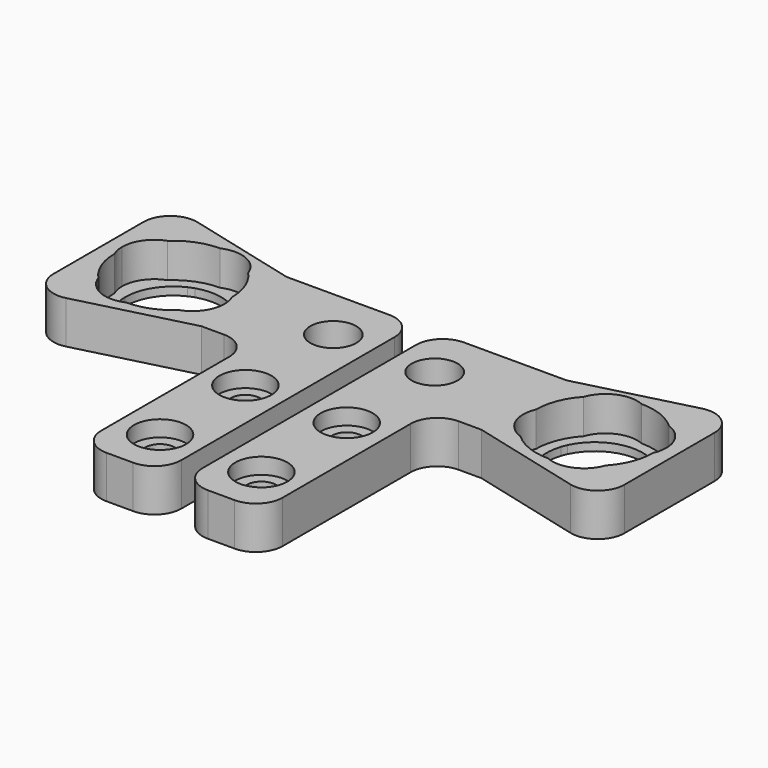
from build123d import *

# Parameters (mm, degrees)
F1_DEPTH       = 8
F2_D           = 8.6
F3_D           = 5.5
F3_CBORE_D     = 9.75
F3_CBORE_DEPTH = 3
F4_R           = 5
F5_START       = -6.5
F5_DEPTH       = 1.5


# Not quite as in the source:
# - a feature names something its author has since deleted; it is built from what else it names


with BuildPart() as f1:
    # F0 (on Top) → F1 (new body)
    with BuildSketch(Plane.XY):
        Polygon((53.5, 33), (53.5, 67), (26.25, 60), (2, 60), (2, 40), (2, 0), (17, 0), (17, 40), (26.25, 40), align=None)
        with BuildLine():
            ThreePointArc((51, 52.3979157617), (50.8736700622, 51.1731708903), (50.5, 50))
            ThreePointArc((50.5, 50), (49.7385612859, 45.978574532), (47.55966131, 42.5138888889))
            ThreePointArc((47.55966131, 42.5138888889), (44.2958315233, 39), (39.5, 39))
            ThreePointArc((39.5, 39), (35.478574532, 39.7614387141), (32.0138888889, 41.94033869))
            ThreePointArc((32.0138888889, 41.94033869), (28.5, 45.2041684767), (28.5, 50))
            ThreePointArc((28.5, 50), (29.2614387141, 54.021425468), (31.44033869, 57.4861111111))
            ThreePointArc((31.44033869, 57.4861111111), (34.7041684767, 61), (39.5, 61))
            ThreePointArc((39.5, 61), (43.521425468, 60.2385612859), (46.9861111111, 58.05966131))
            ThreePointArc((46.9861111111, 58.05966131), (49.8947250519, 55.8680262306), (51, 52.3979157617))
        make_face(mode=Mode.SUBTRACT)
    extrude(amount=-F1_DEPTH)

    # F2 (through all)
    with Locations(Plane.XY):
        with Locations((9.5, 50)):
            Hole(F2_D / 2)

    # F3 (through all)
    with Locations(Plane.XY):
        with Locations((9.5, 29.4), (9.5, 9.4)):
            CounterBoreHole(F3_D / 2, F3_CBORE_D / 2, F3_CBORE_DEPTH)

    # F4
    f4_edges = [f1.edges().sort_by_distance(p)[0] for p in [
        (17, 0, -4),
        (2, 60, -4),
        (53.5, 33, -4),
        (53.5, 67, -4),
        (17, 40, -4),
        (2, 0, -4),
    ]]
    fillet(f4_edges, radius=F4_R)

    # F0 (on Top) → F5 (join)
    with BuildSketch(Plane.XY.offset(F5_START)):
        with BuildLine():
            ThreePointArc((42.2592068472, 58.5666082888), (41.0707112049, 60), (39.5, 61))
            ThreePointArc((39.5, 61), (35.1038211036, 60.0833333333), (31.44033869, 57.4861111111))
            ThreePointArc((31.44033869, 57.4861111111), (31.104078936, 55.6547009803), (31.3454826891, 53.8083917112))
            ThreePointArc((31.3454826891, 53.8083917112), (35.9031263575, 58.25), (42.2592068472, 58.5666082888))
        make_face()
        with BuildLine():
            ThreePointArc((31.44033869, 57.4861111111), (35.1038211036, 60.0833333333), (39.5, 61))
            ThreePointArc((39.5, 61), (34.7041684767, 61), (31.44033869, 57.4861111111))
        make_face()
        with BuildLine():
            ThreePointArc((43.3083917112, 58.1545173109), (45.1547009803, 58.395921064), (46.9861111111, 58.05966131))
            ThreePointArc((46.9861111111, 58.05966131), (43.521425468, 60.2385612859), (39.5, 61))
            ThreePointArc((39.5, 61), (41.0707112049, 60), (42.2592068472, 58.5666082888))
            ThreePointArc((42.2592068472, 58.5666082888), (42.7902572011, 58.3770046885), (43.3083917112, 58.1545173109))
        make_face()
        with BuildLine():
            ThreePointArc((48.0666082888, 47.2407931528), (49.5, 48.4292887951), (50.5, 50))
            ThreePointArc((50.5, 50), (49.5833333333, 54.3961788964), (46.9861111111, 58.05966131))
            ThreePointArc((46.9861111111, 58.05966131), (45.1547009803, 58.395921064), (43.3083917112, 58.1545173109))
            ThreePointArc((43.3083917112, 58.1545173109), (47.0919538131, 54.8334498342), (48.5, 50))
            ThreePointArc((48.5, 50), (48.3909919188, 48.603481937), (48.0666082888, 47.2407931528))
        make_face()
        with BuildLine():
            ThreePointArc((46.9861111111, 58.05966131), (49.5833333333, 54.3961788964), (50.5, 50))
            ThreePointArc((50.5, 50), (50.8736700622, 51.1731708903), (51, 52.3979157617))
            ThreePointArc((51, 52.3979157617), (49.8947250519, 55.8680262306), (46.9861111111, 58.05966131))
        make_face()
        with BuildLine():
            ThreePointArc((47.55966131, 42.5138888889), (49.7385612859, 45.978574532), (50.5, 50))
            ThreePointArc((50.5, 50), (49.5, 48.4292887951), (48.0666082888, 47.2407931528))
            ThreePointArc((48.0666082888, 47.2407931528), (47.8770046885, 46.7097427989), (47.6545173109, 46.1916082888))
            ThreePointArc((47.6545173109, 46.1916082888), (47.8367544232, 45.3545146881), (47.8979157617, 44.5))
            ThreePointArc((47.8979157617, 44.5), (47.8127476819, 43.4926453678), (47.55966131, 42.5138888889))
        make_face()
        with BuildLine():
            ThreePointArc((39.5, 39), (43.8961788964, 39.9166666667), (47.55966131, 42.5138888889))
            ThreePointArc((47.55966131, 42.5138888889), (47.8127476819, 43.4926453678), (47.8979157617, 44.5))
            ThreePointArc((47.8979157617, 44.5), (47.8367544232, 45.3545146881), (47.6545173109, 46.1916082888))
            ThreePointArc((47.6545173109, 46.1916082888), (43.0968736425, 41.75), (36.7407931528, 41.4333917112))
            ThreePointArc((36.7407931528, 41.4333917112), (37.9292887951, 40), (39.5, 39))
        make_face()
        with BuildLine():
            ThreePointArc((39.5, 39), (44.2958315233, 39), (47.55966131, 42.5138888889))
            ThreePointArc((47.55966131, 42.5138888889), (43.8961788964, 39.9166666667), (39.5, 39))
        make_face()
        with BuildLine():
            ThreePointArc((32.0138888889, 41.94033869), (35.478574532, 39.7614387141), (39.5, 39))
            ThreePointArc((39.5, 39), (37.9292887951, 40), (36.7407931528, 41.4333917112))
            ThreePointArc((36.7407931528, 41.4333917112), (36.2097427989, 41.6229953115), (35.6916082888, 41.8454826891))
            ThreePointArc((35.6916082888, 41.8454826891), (33.8452990197, 41.604078936), (32.0138888889, 41.94033869))
        make_face()
        with BuildLine():
            ThreePointArc((28.5, 50), (29.4166666667, 45.6038211036), (32.0138888889, 41.94033869))
            ThreePointArc((32.0138888889, 41.94033869), (33.8452990197, 41.604078936), (35.6916082888, 41.8454826891))
            ThreePointArc((35.6916082888, 41.8454826891), (31.25, 46.4031263575), (30.9333917112, 52.7592068472))
            ThreePointArc((30.9333917112, 52.7592068472), (29.5, 51.5707112049), (28.5, 50))
        make_face()
        with BuildLine():
            ThreePointArc((28.5, 50), (28.5, 45.2041684767), (32.0138888889, 41.94033869))
            ThreePointArc((32.0138888889, 41.94033869), (29.4166666667, 45.6038211036), (28.5, 50))
        make_face()
        with BuildLine():
            ThreePointArc((31.3454826891, 53.8083917112), (31.104078936, 55.6547009803), (31.44033869, 57.4861111111))
            ThreePointArc((31.44033869, 57.4861111111), (29.2614387141, 54.021425468), (28.5, 50))
            ThreePointArc((28.5, 50), (29.5, 51.5707112049), (30.9333917112, 52.7592068472))
            ThreePointArc((30.9333917112, 52.7592068472), (31.1229953115, 53.2902572011), (31.3454826891, 53.8083917112))
        make_face()
    extrude(amount=-F5_DEPTH)


with BuildPart() as f6_1:
    # F6: instance of F1
    add(f1.part.mirror(Plane.YZ))


solid = Compound([f1.part, f6_1.part])
